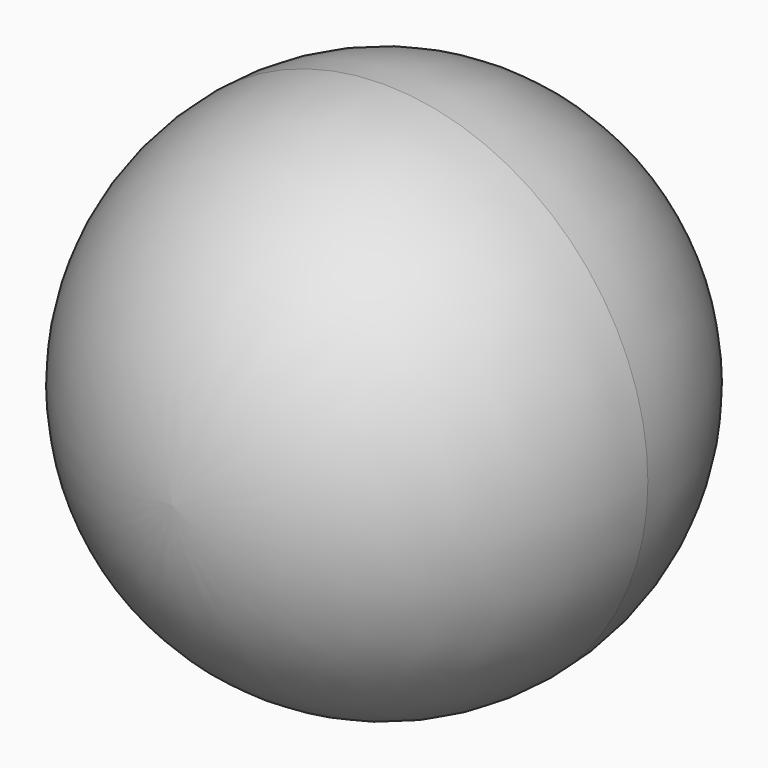
from build123d import *

# Parameters (mm, degrees)
F0_R     = 5.5
F1_DEPTH = 11
F2_R     = 5.49999


# Not quite as in the source:
# - a fillet or chamfer is up to 0.001 mm smaller than in the source, because OpenCascade refuses the exact size


with BuildPart() as f1:
    # F0 (on Front) → F1 (new body)
    with BuildSketch(Plane.XZ):
        Circle(F0_R)
    extrude(amount=F1_DEPTH)

    # F2 (radius 5.5 in the source; OpenCascade refuses exactly that, so slightly less here)
    f2_edges = [f1.edges().sort_by_distance(p)[0] for p in [
        (-5.5, -11, 0),
        (-5.5, 0, 0),
    ]]
    fillet(f2_edges, radius=F2_R)


solid = f1.part
